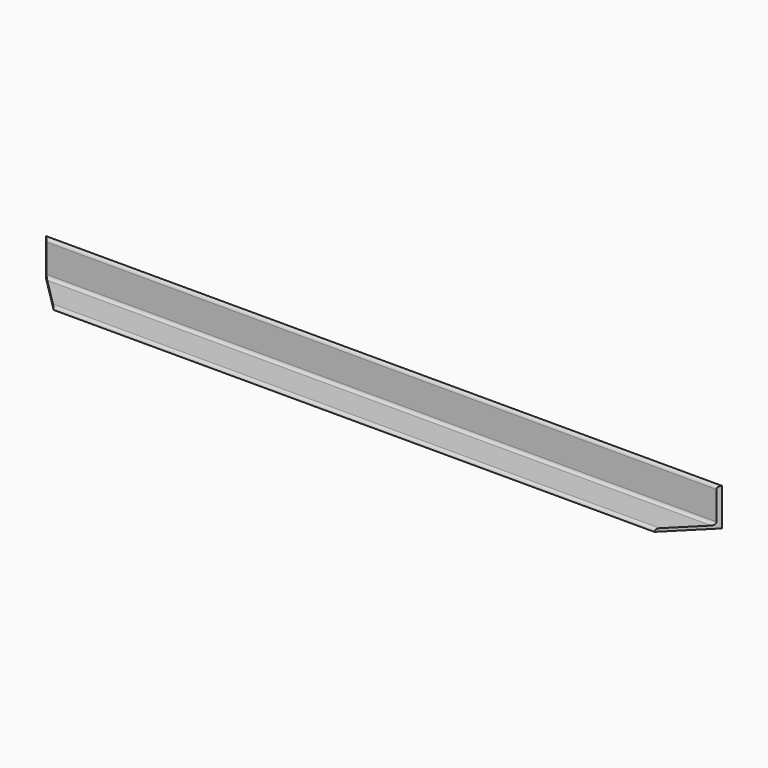
from build123d import *

# Parameters (mm, degrees)
F1_DEPTH = 450
F3_DEPTH = 50.001


# Not quite as in the source:
# - a pattern or mirror of a feature is missing from the dataset's text; its kind, count and spacing are read off the source's solid


with BuildPart() as f1:
    # F0 (on Right) → F1 (new body, symmetric)
    with BuildSketch(Plane.YZ):
        with BuildLine():
            Line((0, 0), (0, 50))
            ThreePointArc((0, 50), (-2.8284271247, 48.8284271247), (-4, 46))
            Line((-4, 46), (-4, 8))
            ThreePointArc((-4, 8), (-5.1715728753, 5.1715728753), (-8, 4))
            Line((-8, 4), (-46, 4))
            ThreePointArc((-46, 4), (-48.8284271247, 2.8284271247), (-50, 0))
            Line((-50, 0), (0, 0))
        make_face()
    extrude(amount=F1_DEPTH, both=True)

    # F2 (on face) → F3 (cut, through all)
    with BuildSketch(Plane(origin=(0, 0, 0), x_dir=(1, 0, 0), z_dir=(0, 0, -1))):
        Polygon((400, 50), (450, 0), (450, 50), align=None)
    f3 = extrude(amount=-F3_DEPTH, mode=Mode.SUBTRACT)

    # F3_copies: F3 across plane
    add(f3.mirror(Plane(origin=(0, 0, 0), x_dir=(0, 0, -1), z_dir=(-1, 0, 0))), mode=Mode.SUBTRACT)


solid = f1.part
